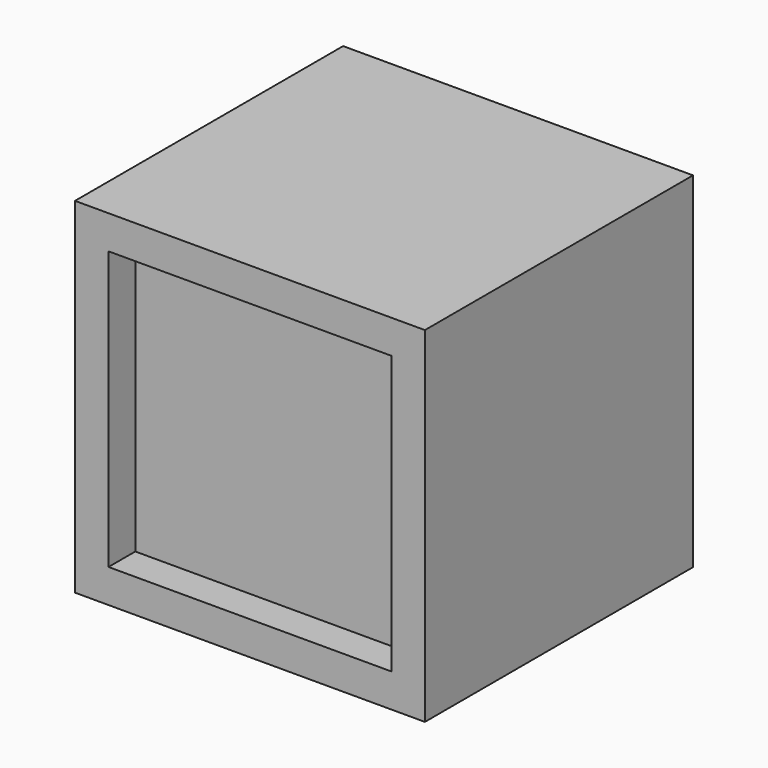
from build123d import *

# Parameters (mm, degrees)
F3_W     = 132.5927376747
F3_H     = 130.7096034288
F4_DEPTH = 127
F0_T     = -12.7
F5_DEPTH = 101.6


# Not quite as in the source:
# - the program builds the solid bodies; features that only make, move or delete a surface that nothing else refers to are left out


with BuildPart() as f4:
    # F3 (on Front) → F4 (new body)
    with BuildSketch(Plane.XZ):
        with Locations((0.488370657, -2.5630220771)):
            Rectangle(F3_W, F3_H)
    extrude(amount=F4_DEPTH)

    # F0
    f0_openings = [f4.faces().sort_by_distance(p)[0] for p in [
        (0.488371, -127, -2.563022),
    ]]
    offset(amount=F0_T, openings=f0_openings)

    # F5 (add): a face of the model
    f5_faces = [f4.faces().sort_by_distance(p)[0] for p in [
        (0.488370657, -12.7, -2.5630220771),
    ]]
    extrude(f5_faces, amount=F5_DEPTH)


solid = f4.part
